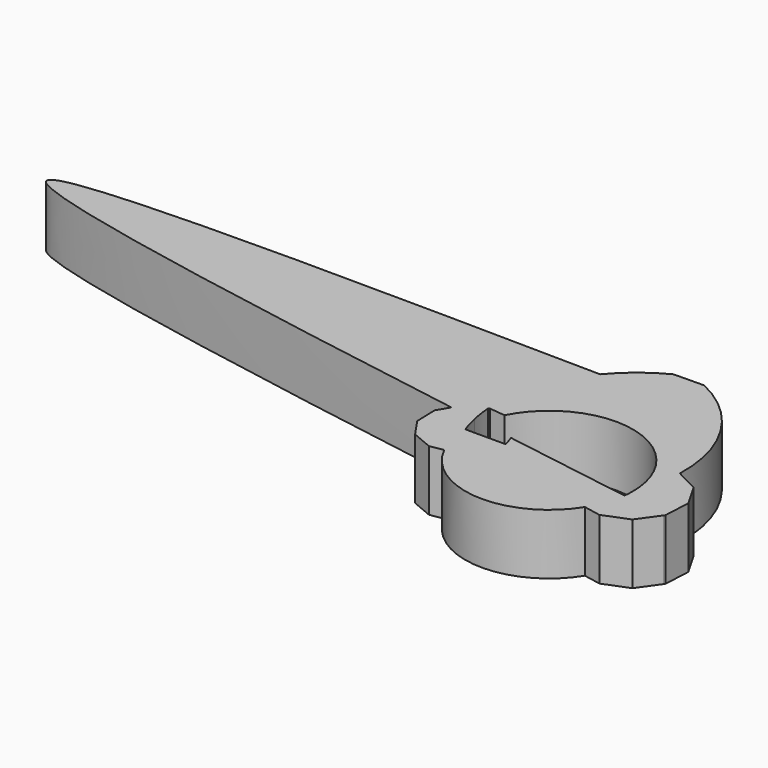
from build123d import *

# Parameters (mm, degrees)
F1_DEPTH    = 25.4
F2_DEPTH    = 25.4
F3_T1_DEPTH = 60.9890887747


# Not quite as in the source:
# - a fillet or chamfer that OpenCascade refuses, or shapes differently, is made with other operations: its cross-section is extruded or revolved along the edge and cut away or added


with BuildPart() as f1:
    # F0 (on Top) → F1 (new body)
    with BuildSketch(Plane.XY):
        with BuildLine():
            Line((0, 0), (9.0822612578, 0))
            add(Edge.make_bspline(
                [(9.0822612578, 0), (-0.5887823283, 1.5524321895), (-10.1972217153, 3.0991138841), (-19.7038336111, 4.636442237)],
                knots=[0.053890232, 0.053890232, 0.053890232, 0.053890232, 0.0876539783, 0.0876539783, 0.0876539783, 0.0876539783], degree=3))
            Line((-19.7038336111, 4.636442237), (-18.3546670651, 0.4999203421))
            Line((-18.3546670651, 0.4999203421), (-18.4854740521, 0))
            Line((-18.4854740521, 0), (0, 0))
        make_face()
    extrude(amount=F1_DEPTH)

    # F0 (on Top) → F2 (join)
    with BuildSketch(Plane.XY):
        with BuildLine():
            ThreePointArc((39.2946183394, 19.5425995517), (38.0990536847, 9.5917687024), (35.1927875929, 0))
            ThreePointArc((35.1927875929, 0), (35.1315324061, -2.0755070121), (34.9479800825, -4.1437889318))
            add(Edge.make_bspline(
                [(53.7340444048, -7.1471543317), (47.4674866948, -6.1456158537), (41.202016032, -5.1441772263), (34.9479800825, -4.1437889318)],
                knots=[0.0022748674, 0.0022748674, 0.0022748674, 0.0022748674, 0.0239294634, 0.0239294634, 0.0239294634, 0.0239294634], degree=3))
            Line((53.7340444048, -7.1471543317), (54.1296049181, -6.5938649088))
            Line((54.1296049181, -6.5938649088), (54.6883645828, 4.6909042491))
            Line((54.6883645828, 4.6909042491), (49.0574163024, 14.4863444523))
            Line((49.0574163024, 14.4863444523), (39.2946183394, 19.5425995517))
        make_face()
        with BuildLine():
            ThreePointArc((29.7418780254, 18.8136384064), (33.8026026699, 9.793689361), (35.1927875929, 0))
            ThreePointArc((35.1927875929, 0), (38.0990536847, 9.5917687024), (39.2946183394, 19.5425995517))
            Line((39.2946183394, 19.5425995517), (39.0245463695, 19.6824726475))
            Line((39.0245463695, 19.6824726475), (29.7418780254, 18.8136384064))
        make_face()
        with BuildLine():
            ThreePointArc((-31.426870984, 15.839320652), (-1.7092225846, 35.1512568298), (29.7418780254, 18.8136384064))
            Line((29.7418780254, 18.8136384064), (39.0245463695, 19.6824726475))
            Line((39.0245463695, 19.6824726475), (39.2946183394, 19.5425995517))
            ThreePointArc((39.2946183394, 19.5425995517), (29.0039385515, 54.2539705519), (0, 75.9230479598))
            ThreePointArc((0, 75.9230479598), (-13.7345779986, 68.6878764709), (-25.1210674885, 58.1363743803))
            ThreePointArc((-25.1210674885, 58.1363743803), (-35.8950760367, 38.527599561), (-38.637588859, 16.3226016208))
            Line((-38.637588859, 16.3226016208), (-38.0839338665, 16.5955866568))
            Line((-38.0839338665, 16.5955866568), (-31.426870984, 15.839320652))
        make_face()
        with BuildLine():
            add(Edge.make_bspline(
                [(53.7340444048, -7.1471543317), (47.4674866948, -6.1456158537), (41.202016032, -5.1441772263), (34.9479800825, -4.1437889318)],
                knots=[0.0022748674, 0.0022748674, 0.0022748674, 0.0022748674, 0.0239294634, 0.0239294634, 0.0239294634, 0.0239294634], degree=3))
            ThreePointArc((34.9479800825, -4.1437889318), (33.2140769684, -11.6343194773), (29.8948841627, -18.56955033))
            Line((29.8948841627, -18.56955033), (37.0614353142, -19.964725406))
            Line((37.0614353142, -19.964725406), (47.5585395538, -15.7851285483))
            Line((47.5585395538, -15.7851285483), (53.7340444048, -7.1471543317))
        make_face()
        with BuildLine():
            ThreePointArc((29.8948841627, -18.56955033), (33.2140769684, -11.6343194773), (34.9479800825, -4.1437889318))
            add(Edge.make_bspline(
                [(34.9479800825, -4.1437889318), (28.5019841788, -3.1126949471), (22.0681357101, -2.0827167623), (15.6577647144, -1.0548950957)],
                knots=[0.0239294634, 0.0239294634, 0.0239294634, 0.0239294634, 0.0462487206, 0.0462487206, 0.0462487206, 0.0462487206], degree=3))
            Line((15.6577647144, -1.0548950956), (17.8084989026, -9.9934284194))
            Line((17.8084989026, -9.9934284194), (25.9710486263, -17.8056630113))
            Line((25.9710486263, -17.8056630113), (29.8948841627, -18.56955033))
        make_face()
        with BuildLine():
            ThreePointArc((-31.4678779331, -15.7576951661), (-1.6109654608, -35.1558969285), (29.8948841627, -18.56955033))
            Line((29.8948841627, -18.56955033), (25.9710486263, -17.8056630113))
            Line((25.9710486263, -17.8056630113), (17.8084989026, -9.9934284194))
            Line((17.8084989026, -9.9934284194), (15.6577647144, -1.0548950956))
            add(Edge.make_bspline(
                [(15.6577647144, -1.0548950957), (13.4630266479, -0.7029966893), (11.271040594, -0.3513510685), (9.0822612578, 0)],
                knots=[0.0462487206, 0.0462487206, 0.0462487206, 0.0462487206, 0.053890232, 0.053890232, 0.053890232, 0.053890232], degree=3))
            Line((9.0822612578, 0), (0, 0))
            Line((0, 0), (-18.4854740521, 0))
            Line((-18.4854740521, 0), (-20.7573818702, -8.6828154927))
            Line((-20.7573818702, -8.6828154927), (-27.7432359966, -15.1088187584))
            Line((-27.7432359966, -15.1088187584), (-31.4678779331, -15.7576951661))
        make_face()
        with BuildLine():
            Line((-37.0942701188, -16.7378788221), (-31.4678779331, -15.7576951661))
            ThreePointArc((-31.4678779331, -15.7576951661), (-34.2489024836, -8.0959852539), (-35.1927875929, 0))
            ThreePointArc((-35.1927875929, 0), (-36.4082086965, 3.7156215634), (-37.3761939959, 7.5032456896))
            add(Edge.make_bspline(
                [(-37.3761939959, 7.5032456896), (-41.0895221285, 8.1076779871), (-44.782988486, 8.7102858856), (-48.4541472769, 9.3108447276)],
                knots=[0.1087279171, 0.1087279171, 0.1087279171, 0.1087279171, 0.1221167407, 0.1221167407, 0.1221167407, 0.1221167407], degree=3))
            Line((-48.4541472769, 9.3108447276), (-51.4896897645, 4.2641766931))
            Line((-51.4896897645, 4.2641766931), (-51.2080020921, -5.2235168043))
            Line((-51.2080020921, -5.2235168043), (-45.8415969743, -13.052780624))
            Line((-45.8415969743, -13.052780624), (-37.0942701188, -16.7378788221))
        make_face()
        with BuildLine():
            ThreePointArc((-35.1927875929, 0), (-34.2489024836, -8.0959852539), (-31.4678779331, -15.7576951661))
            Line((-31.4678779331, -15.7576951661), (-27.7432359966, -15.1088187584))
            Line((-27.7432359966, -15.1088187584), (-20.7573818702, -8.6828154927))
            Line((-20.7573818702, -8.6828154927), (-18.4854740521, 0))
            Line((-18.4854740521, 0), (-35.1927875929, 0))
        make_face()
        with BuildLine():
            ThreePointArc((-38.637588859, 16.3226016208), (-35.8950760367, 38.527599561), (-25.1210674885, 58.1363743803))
            add(Edge.make_bspline(
                [(-48.4541472769, 9.3108447276), (-161.5048500043, 27.8046236609), (-354.0298848729, 62.4785632102), (-140.2321873005, 59.829817618), (-25.1210674885, 58.1363743803)],
                knots=[0.1221167407, 0.1221167407, 0.1221167407, 0.1221167407, 0.5344159633, 0.9858900342, 0.9858900342, 0.9858900342, 0.9858900342], degree=3))
            Line((-48.4541472769, 9.3108447276), (-46.5972261458, 12.3980242197))
            Line((-46.5972261458, 12.3980242197), (-38.637588859, 16.3226016208))
        make_face()
        with BuildLine():
            add(Edge.make_bspline(
                [(-37.3761939959, 7.5032456896), (-41.0895221285, 8.1076779871), (-44.782988486, 8.7102858856), (-48.4541472769, 9.3108447276)],
                knots=[0.1087279171, 0.1087279171, 0.1087279171, 0.1087279171, 0.1221167407, 0.1221167407, 0.1221167407, 0.1221167407], degree=3))
            ThreePointArc((-37.3761939959, 7.5032456896), (-38.172734201, 11.8892038706), (-38.637588859, 16.3226016208))
            Line((-38.637588859, 16.3226016208), (-46.5972261458, 12.3980242197))
            Line((-46.5972261458, 12.3980242197), (-48.4541472769, 9.3108447276))
        make_face()
    extrude(amount=F2_DEPTH)

    # F3: chamfer of 5.08 on 1 edges, made by hand

    # F3_s2 → F3_t1 (cut)
    with BuildSketch(Plane.XY.offset(-17.7945443873)):
        with BuildLine():
            Line((6.6348201683, 73.3457449263), (-6.5209439135, 73.161183328))
            Line((-6.5209439135, 73.161183328), (-6.5669480575, 73.2517712893))
            ThreePointArc((-6.5669480575, 73.2517712893), (-3.3257137482, 74.6908686941), (-0.0351808653, 76.018362527))
            Line((-0.0351808653, 76.018362527), (0.0320735811, 76.019452552))
            ThreePointArc((0.0320735811, 76.019452552), (3.3798158566, 74.7892252054), (6.6782649991, 73.4375877631))
            Line((6.6782649991, 73.4375877631), (6.6348201683, 73.3457449263))
        make_face()
    extrude(amount=F3_T1_DEPTH, mode=Mode.SUBTRACT)


solid = f1.part
